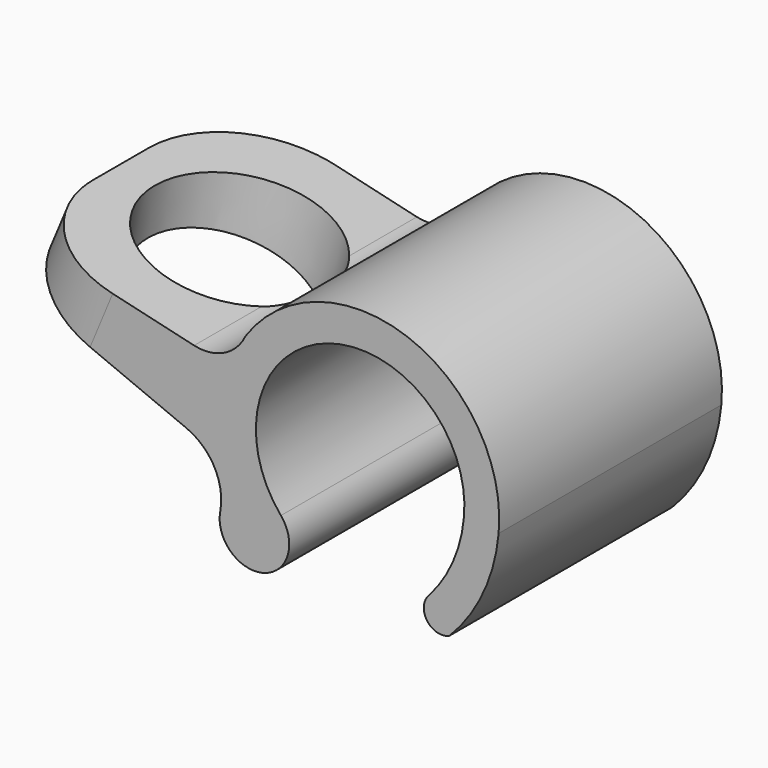
from build123d import *

# Parameters (mm, degrees)
F1_DEPTH      = 25.4
F2_R          = 7.9375
F3_DEPTH      = 25.4
F3_TAPER      = 5
F3_DEPTH_BACK = 25.4
F4_R          = 9.525


with BuildPart() as f1:
    # F0 (on Front) → F1 (new body)
    with BuildSketch(Plane.XZ):
        with BuildLine():
            ThreePointArc((15.9420039577, -5.3261326592), (14.9211079736, -9.2769096997), (12.7, -12.7))
            ThreePointArc((12.7, -12.7), (12.5948783029, -14.7822408301), (14.6158441263, -15.2945635671))
            ThreePointArc((14.6158441263, -15.2945635671), (17.697106564, -10.8437100374), (19.1037159776, -5.6163086455))
            ThreePointArc((19.1037159776, -5.6163086455), (10.77478978, 7.4777303194), (-3.9952923544, 2.7164760977))
            ThreePointArc((-3.9952923544, 2.7164760977), (-5.934088224, 0.7499909222), (-8.6788133112, 0.4458896807))
            Line((-8.6788133112, 0.4458896807), (-25.5047661099, 4.3984803395))
            Line((-25.5047661099, 4.3984803395), (-26.9643777894, 0.8821428277))
            Line((-26.9643777894, 0.8821428277), (-9.3699563909, -6.421201314))
            ThreePointArc((-9.3699563909, -6.421201314), (-6.8229957257, -8.720792311), (-6.2949665087, -12.1114135711))
            ThreePointArc((-6.2949665087, -12.1114135711), (-2.3576029431, -15.767977681), (-0.7614577713, -10.6371284795))
            ThreePointArc((-0.7614577713, -10.6371284795), (3.5871947735, 4.6083370701), (15.9420039577, -5.3261326592))
        make_face()
    extrude(amount=F1_DEPTH)

    # F2 (on face) → F3 (cut, two sides)
    with BuildSketch(Plane(origin=(-0.354609422, 0, -1.5095520662), x_dir=(0.9735003954, 0, -0.22868533), z_dir=(0.22868533, 0, 0.9735003954))) as f3_sk:
        with Locations((-14.7222678204, -12.7)):
            Circle(F2_R)
    extrude(amount=-F3_DEPTH, taper=F3_TAPER, mode=Mode.SUBTRACT)
    extrude(f3_sk.sketch, amount=F3_DEPTH_BACK, mode=Mode.SUBTRACT)

    # F4
    f4_edges = [f1.edges().sort_by_distance(p)[0] for p in [
        (-26.234572, 0, 2.640312),
        (-26.234572, -25.4, 2.640312),
    ]]
    fillet(f4_edges, radius=F4_R)


solid = f1.part
